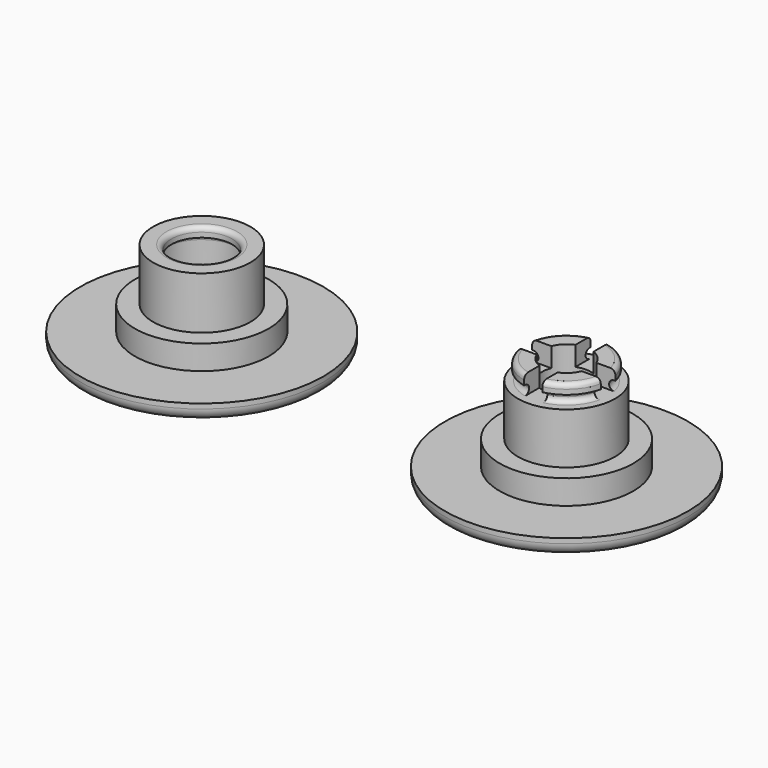
from build123d import *

# Parameters (mm, degrees)
F0_R      = 10
F1_DEPTH  = 1.4
F2_R      = 5.5
F3_DEPTH  = 2
F5_R      = 4
F5_R_2    = 3
F6_DEPTH  = 3.5
F7_R      = 4
F7_R_2    = 3
F7_R_3    = 2.5
F8_DEPTH  = 0.8
F9_R      = 4
F9_R_2    = 2
F10_DEPTH = 4.2
F11_R     = 3
F11_R_2   = 2
F12_DEPTH = 0.8
F13_R     = 3.5
F13_R_2   = 3
F13_R_3   = 2
F14_DEPTH = 0.8
F15_R     = 1
F15_2_R   = 1
F16_R     = 0.39999
F16_2_R   = 0.39999
F18_DEPTH = 1.6


# Not quite as in the source:
# - a fillet or chamfer is up to 0.001 mm smaller than in the source, because OpenCascade refuses the exact size


with BuildPart() as f1:
    # F0 (on Top) → F1 (new body)
    with BuildSketch(Plane.XY):
        Circle(F0_R)
    extrude(amount=F1_DEPTH)

    # F2 (on face) → F3 (join)
    with BuildSketch(Plane.XY.offset(1.4)):
        Circle(F2_R)
    extrude(amount=F3_DEPTH)


with BuildPart() as f4_1:
    # F4: copy of F1
    add(f1.part.moved(Location((30, 0, 0))))

    # F9 (on face) → F10 (join)
    with BuildSketch(Plane.XY.offset(3.4)):
        with Locations((30, 0)):
            Circle(F9_R)
        with Locations((30, 0)):
            Circle(F9_R_2, mode=Mode.SUBTRACT)
    extrude(amount=F10_DEPTH)

    # F11 (on face) → F12 (join)
    with BuildSketch(Plane.XY.offset(7.6)):
        with Locations((30, 0)):
            Circle(F11_R)
        with Locations((30, 0)):
            Circle(F11_R_2, mode=Mode.SUBTRACT)
    extrude(amount=F12_DEPTH)

    # F13 (on face) → F14 (join)
    with BuildSketch(Plane.XY.offset(8.4)):
        with Locations((30, 0)):
            Circle(F13_R)
        with Locations((30, 0)):
            Circle(F13_R_2, mode=Mode.SUBTRACT)
        with Locations((30, 0)):
            Circle(F13_R_2)
        with Locations((30, 0)):
            Circle(F13_R_3, mode=Mode.SUBTRACT)
    extrude(amount=F14_DEPTH)

    # F15#2
    f15_2_edges = [f4_1.edges().sort_by_distance(p)[0] for p in [
        (20, 0, 0),
    ]]
    fillet(f15_2_edges, radius=F15_2_R)

    # F16 (radius 0.4 in the source; OpenCascade refuses exactly that, so slightly less here)
    f16_edges = [f4_1.edges().sort_by_distance(p)[0] for p in [
        (26.5, 0, 9.2),
        (27, 0, 8.4),
        (27, 0, 7.6),
    ]]
    fillet(f16_edges, radius=F16_R)

    # F17 (on face) → F18 (cut, through all)
    with BuildSketch(Plane.XY.offset(9.2)):
        with BuildLine():
            Line((30.75, 1.8540496218), (30.75, 3.0079165547))
            ThreePointArc((30.75, 3.0079165547), (30, 3.10001), (29.25, 3.0079165547))
            Line((29.25, 3.0079165547), (29.25, 1.8540496218))
            ThreePointArc((29.25, 1.8540496218), (30, 2), (30.75, 1.8540496218))
        make_face()
        with BuildLine():
            Line((30.75, 0.75), (30.75, 1.8540496218))
            ThreePointArc((30.75, 1.8540496218), (30, 2), (29.25, 1.8540496218))
            Line((29.25, 1.8540496218), (29.25, 0.75))
            Line((29.25, 0.75), (28.1459503782, 0.75))
            ThreePointArc((28.1459503782, 0.75), (28, 0), (28.1459503782, -0.75))
            Line((28.1459503782, -0.75), (29.25, -0.75))
            Line((29.25, -0.75), (29.25, -1.8540496218))
            ThreePointArc((29.25, -1.8540496218), (30, -2), (30.75, -1.8540496218))
            Line((30.75, -1.8540496218), (30.75, -0.75))
            Line((30.75, -0.75), (31.8540496218, -0.75))
            ThreePointArc((31.8540496218, -0.75), (31.963173355, -0.3820345249), (32, 0))
            ThreePointArc((32, 0), (31.963173355, 0.3820345249), (31.8540496218, 0.75))
            Line((31.8540496218, 0.75), (30.75, 0.75))
        make_face()
        with BuildLine():
            ThreePointArc((33.10001, 0), (33.076900502, 0.3778164907), (33.0079165547, 0.75))
            Line((33.0079165547, 0.75), (31.8540496218, 0.75))
            ThreePointArc((31.8540496218, 0.75), (31.963173355, 0.3820345249), (32, 0))
            ThreePointArc((32, 0), (31.963173355, -0.3820345249), (31.8540496218, -0.75))
            Line((31.8540496218, -0.75), (33.0079165547, -0.75))
            ThreePointArc((33.0079165547, -0.75), (33.076900502, -0.3778164907), (33.10001, 0))
        make_face()
        with BuildLine():
            Line((29.25, -1.8540496218), (29.25, -3.0079165547))
            ThreePointArc((29.25, -3.0079165547), (30, -3.10001), (30.75, -3.0079165547))
            Line((30.75, -3.0079165547), (30.75, -1.8540496218))
            ThreePointArc((30.75, -1.8540496218), (30, -2), (29.25, -1.8540496218))
        make_face()
        with BuildLine():
            Line((28.1459503782, 0.75), (26.9920834453, 0.75))
            ThreePointArc((26.9920834453, 0.75), (26.89999, 0), (26.9920834453, -0.75))
            Line((26.9920834453, -0.75), (28.1459503782, -0.75))
            ThreePointArc((28.1459503782, -0.75), (28, 0), (28.1459503782, 0.75))
        make_face()
        with BuildLine():
            Line((36.5956649214, 0.75), (33.0079165547, 0.75))
            ThreePointArc((33.0079165547, 0.75), (33.076900502, 0.3778164907), (33.10001, 0))
            ThreePointArc((33.10001, 0), (33.076900502, -0.3778164907), (33.0079165547, -0.75))
            Line((33.0079165547, -0.75), (36.5956649214, -0.75))
            Line((36.5956649214, -0.75), (36.5956649214, 0.75))
        make_face()
        with BuildLine():
            ThreePointArc((30.75, -3.0079165547), (30, -3.10001), (29.25, -3.0079165547))
            Line((29.25, -3.0079165547), (29.25, -7.5652996811))
            Line((29.25, -7.5652996811), (30.75, -7.5652996811))
            Line((30.75, -7.5652996811), (30.75, -3.0079165547))
        make_face()
        with BuildLine():
            ThreePointArc((26.9920834453, -0.75), (26.89999, 0), (26.9920834453, 0.75))
            Line((26.9920834453, 0.75), (23.4043350786, 0.75))
            Line((23.4043350786, 0.75), (23.4043350786, -0.75))
            Line((23.4043350786, -0.75), (26.9920834453, -0.75))
        make_face()
        with BuildLine():
            Line((30.75, 3.0079165547), (30.75, 7.5652996811))
            Line((30.75, 7.5652996811), (29.25, 7.5652996811))
            Line((29.25, 7.5652996811), (29.25, 3.0079165547))
            ThreePointArc((29.25, 3.0079165547), (30, 3.10001), (30.75, 3.0079165547))
        make_face()
    extrude(amount=-F18_DEPTH, mode=Mode.SUBTRACT)


with BuildPart() as f1_1:
    add(f1.part)

    # F5 (on face) → F6 (join)
    with BuildSketch(Plane.XY.offset(3.4)):
        Circle(F5_R)
        Circle(F5_R_2, mode=Mode.SUBTRACT)
    extrude(amount=F6_DEPTH)

    # F7 (on face) → F8 (join)
    with BuildSketch(Plane.XY.offset(6.9)):
        Circle(F7_R)
        Circle(F7_R_2, mode=Mode.SUBTRACT)
        Circle(F7_R_2)
        Circle(F7_R_3, mode=Mode.SUBTRACT)
    extrude(amount=F8_DEPTH)

    # F15
    f15_edges = [f1_1.edges().sort_by_distance(p)[0] for p in [
        (-10, 0, 0),
    ]]
    fillet(f15_edges, radius=F15_R)

    # F16#2 (radius 0.4 in the source; OpenCascade refuses exactly that, so slightly less here)
    f16_2_edges = [f1_1.edges().sort_by_distance(p)[0] for p in [
        (-2.5, 0, 7.7),
        (-3, 0, 6.9),
    ]]
    fillet(f16_2_edges, radius=F16_2_R)


solid = Compound([f4_1.part, f1_1.part])
